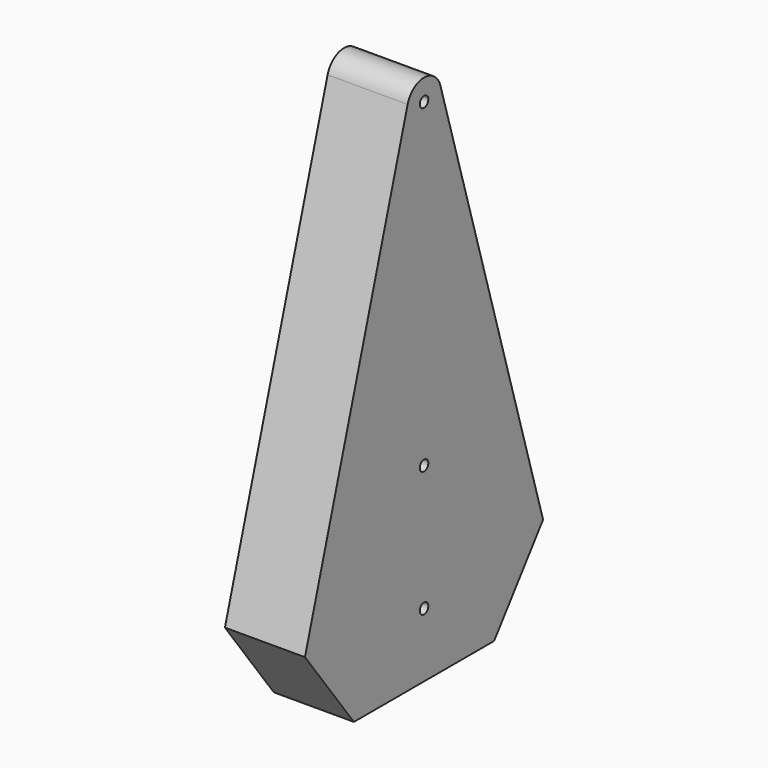
from build123d import *

# Parameters (mm, degrees)
F0_R     = 5
F1_DEPTH = 75
F2_SIZE  = 80


# Not quite as in the source:
# - a feature names something its author has since deleted; it is built from what else it names


with BuildPart() as f1:
    # F0 (on Right) → F1 (new body)
    with BuildSketch(Plane.YZ):
        with BuildLine():
            Line((162.1119900143, -178.1254678004), (19.1804298411, 305.6666666667))
            ThreePointArc((19.1804298411, 305.6666666667), (0, 320), (-19.1804298411, 305.6666666667))
            Line((-19.1804298411, 305.6666666667), (-162.1119900143, -178.1254678004))
            Line((-162.1119900143, -178.1254678004), (162.1119900143, -178.1254678004))
        make_face()
        with Locations((0, -117.917008698)):
            Circle(F0_R, mode=Mode.SUBTRACT)
        Circle(F0_R, mode=Mode.SUBTRACT)
        with Locations((0, 300)):
            Circle(F0_R, mode=Mode.SUBTRACT)
    extrude(amount=F1_DEPTH)

    # F2
    f2_edges = [f1.edges().sort_by_distance(p)[0] for p in [
        (37.5, 162.11199, -178.125468),
        (37.5, -162.11199, -178.125468),
    ]]
    chamfer(f2_edges, length=F2_SIZE)


solid = f1.part
